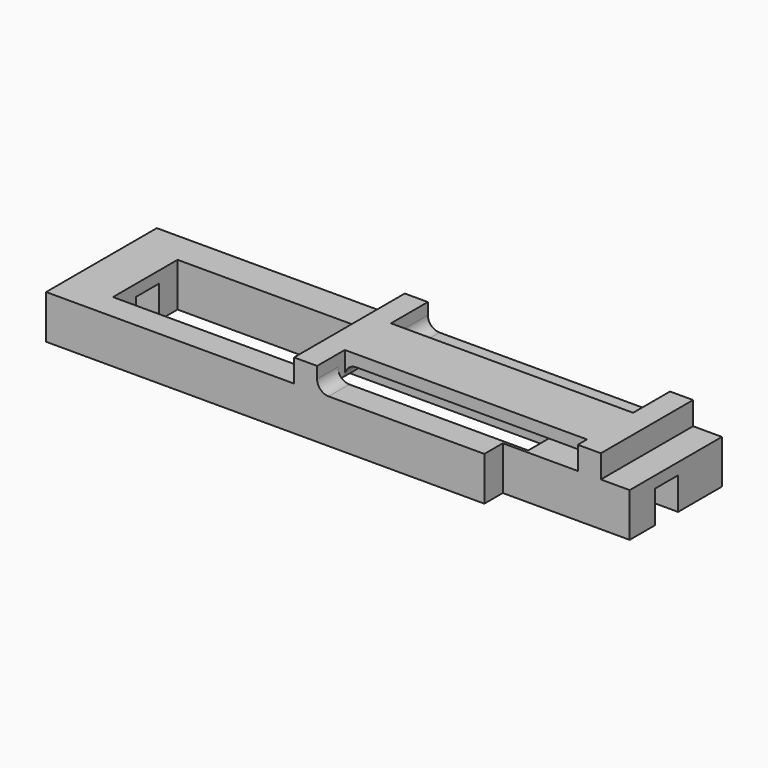
from build123d import *

# Parameters (mm, degrees)
F0_W     = 30
F0_H     = 12
F0_W_2   = 19
F1_DEPTH = 3.8
F2_W     = 1.9557817429
F2_H     = 2.5
F2_W_2   = 17.5
F2_H_2   = 2
F2_W_3   = 2
F2_W_4   = 16.5
F2_W_5   = 4.5
F2_W_6   = 2.5
F2_W_7   = 2.0442182571
F3_DEPTH = 25
F4_DEPTH = 1
F2_H_3   = 2.75
F2_H_4   = 2.25
F2_H_5   = 4.75
F2_H_6   = 0.25
F5_DEPTH = 2
F6_W     = 21
F6_H     = 5
F6_R     = 1
F7_DEPTH = 1
F8_DEPTH = 2
F9_R     = 0.99999


# Not quite as in the source:
# - a fillet or chamfer is up to 0.001 mm smaller than in the source, because OpenCascade refuses the exact size


with BuildPart() as f1:
    # F0 (on Top) → F1 (new body)
    with BuildSketch(Plane.XY):
        with Locations((15, -6)):
            Rectangle(F0_W, F0_H)
        with Locations((-9.5, -6)):
            Rectangle(F0_W_2, F0_H)
    extrude(amount=F1_DEPTH)

    # F2 (on face) → F3 (cut)
    with BuildSketch(Plane.XY.offset(3.8)):
        with Locations((-18.0221091285, -6)):
            Rectangle(F2_W, F2_H)
        with Locations((-6.25, -3.75)):
            Rectangle(F2_W_2, F2_H_2)
        with Locations((-6.25, -6)):
            Rectangle(F2_W_2, F2_H)
        with Locations((-6.25, -8.5)):
            Rectangle(F2_W_2, F2_H)
        with Locations((3.5, -3.75)):
            Rectangle(F2_W_3, F2_H_2)
        with Locations((3.5, -6)):
            Rectangle(F2_W_3, F2_H)
        with Locations((3.5, -8.5)):
            Rectangle(F2_W_3, F2_H)
        with Locations((12.75, -8.5)):
            Rectangle(F2_W_4, F2_H)
        with Locations((12.75, -6)):
            Rectangle(F2_W_4, F2_H)
        with Locations((12.75, -3.75)):
            Rectangle(F2_W_4, F2_H_2)
        with Locations((23.25, -6)):
            Rectangle(F2_W_5, F2_H)
        with Locations((26.5, -6)):
            Rectangle(F2_W_3, F2_H)
        with Locations((28.75, -6)):
            Rectangle(F2_W_6, F2_H)
        Polygon((19, -12), (30, -12), (30, -10), (27.5, -10), (25.5, -10), (19, -10), align=None)
        with Locations((-16.0221091285, -6)):
            Rectangle(F2_W_7, F2_H)
    extrude(amount=-F3_DEPTH, mode=Mode.SUBTRACT)

    # F2 (on face) → F4 (join)
    with BuildSketch(Plane.XY.offset(3.8)):
        with Locations((-18.0221091285, -6)):
            Rectangle(F2_W, F2_H)
        with Locations((23.25, -6)):
            Rectangle(F2_W_5, F2_H)
        with Locations((26.5, -6)):
            Rectangle(F2_W_3, F2_H)
        with Locations((28.75, -6)):
            Rectangle(F2_W_6, F2_H)
        with Locations((-16.0221091285, -6)):
            Rectangle(F2_W_7, F2_H)
    extrude(amount=-F4_DEPTH)

    # F2 (on face) → F5 (join)
    with BuildSketch(Plane.XY.offset(3.8)):
        with Locations((3.5, -1.375)):
            Rectangle(F2_W_3, F2_H_3)
        with Locations((3.5, -3.75)):
            Rectangle(F2_W_3, F2_H_2)
        with Locations((3.5, -6)):
            Rectangle(F2_W_3, F2_H)
        with Locations((3.5, -8.5)):
            Rectangle(F2_W_3, F2_H)
        with Locations((3.5, -10.875)):
            Rectangle(F2_W_3, F2_H_4)
        with Locations((26.5, -2.375)):
            Rectangle(F2_W_3, F2_H_5)
        with Locations((26.5, -6)):
            Rectangle(F2_W_3, F2_H)
        with Locations((26.5, -8.5)):
            Rectangle(F2_W_3, F2_H)
        with Locations((26.5, -9.875)):
            Rectangle(F2_W_3, F2_H_6)
    extrude(amount=F5_DEPTH)

    # F6 (on face) → F7 (join)
    with BuildSketch(Plane.XY.offset(5.8)):
        with Locations((15, -6.5)):
            Rectangle(F6_W, F6_H)
        with Locations((12.75, -6.5)):
            Circle(F6_R, mode=Mode.SUBTRACT)
    extrude(amount=-F7_DEPTH)

    # F6 (on face) → F8 (join)
    with BuildSketch(Plane.XY.offset(5.8)):
        with Locations((12.75, -6.5)):
            Circle(F6_R)
    extrude(amount=-F8_DEPTH)

    # F9 (radius 1 in the source; OpenCascade refuses exactly that, so slightly less here)
    f9_edges = [f1.edges().sort_by_distance(p)[0] for p in [
        (11.75, -6.5, 3.8),
        (25.5, -6.5, 4.8),
        (4.5, -6.5, 4.8),
        (4.5, -10.875, 3.8),
        (4.5, -1.375, 3.8),
    ]]
    fillet(f9_edges, radius=F9_R)


solid = f1.part
